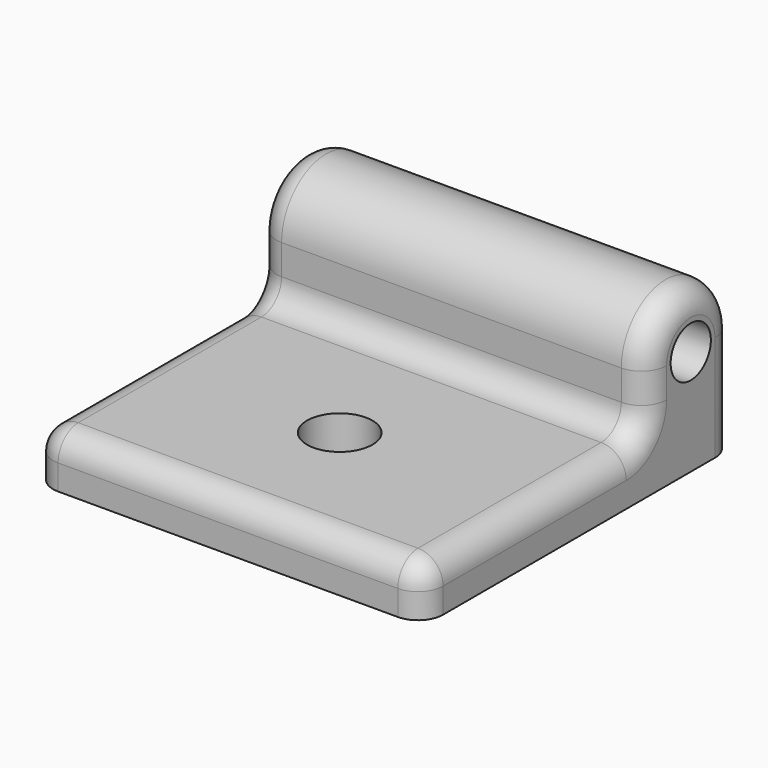
from build123d import *

# Parameters (mm, degrees)
F0_W     = 31
F0_H     = 8.8
F0_H_2   = 22.2
F0_R     = 2.6
F1_DEPTH = 4
F2_DEPTH = 4.4
F3_W     = 31
F3_H     = 4.4
F5_R     = 2
F6_DEPTH = 31.001
F7_R     = 2


with BuildPart() as f1:
    # F0 (on Top) → F1 (new body)
    with BuildSketch(Plane.XY):
        with Locations((-56.2723039389, 48.8844518721)):
            Rectangle(F0_W, F0_H)
        with Locations((-56.2723039389, 33.3844518721)):
            Rectangle(F0_W, F0_H_2)
        with Locations((-56.2723039389, 33.3844518721)):
            Circle(F0_R, mode=Mode.SUBTRACT)
    extrude(amount=-F1_DEPTH)

    # F0 (on Top) → F2 (join)
    with BuildSketch(Plane.XY):
        with Locations((-56.2723039389, 48.8844518721)):
            Rectangle(F0_W, F0_H)
    extrude(amount=F2_DEPTH)

    # F3 (on face) → F4 (revolve)
    with BuildSketch(Plane.XY.offset(4.4)):
        with Locations((-56.2723039389, 46.6844518721)):
            Rectangle(F3_W, F3_H)
    revolve(axis=Axis((-56.2723039389, 48.8844518721, 4.4), (-1, 0, 0)))

    # F5 (on face) → F6 (cut, through all)
    with BuildSketch(Plane.YZ.offset(-40.7723039389)):
        with Locations((48.8844518721, 4.4)):
            Circle(F5_R)
    extrude(amount=-F6_DEPTH, mode=Mode.SUBTRACT)

    # F7
    f7_edges = [f1.edges().sort_by_distance(p)[0] for p in [
        (-56.272304, 44.484452, 0),
        (-40.772304, 22.284452, -2),
        (-71.772304, 22.284452, -2),
        (-56.272304, 22.284452, 0),
        (-40.772304, 33.384452, 0),
        (-71.772304, 33.384452, 0),
        (-71.772304, 53.284452, 0.2),
        (-40.772304, 53.284452, 0.2),
        (-71.772304, 48.884452, 8.8),
        (-40.772304, 48.884452, 8.8),
    ]]
    fillet(f7_edges, radius=F7_R)


solid = f1.part
